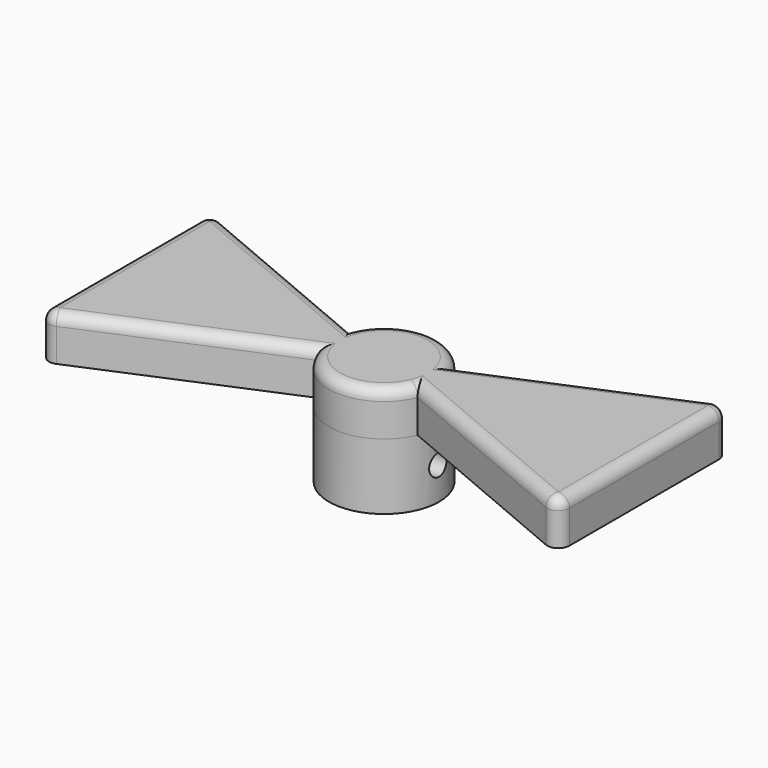
from build123d import *

# Parameters (mm, degrees)
F1_DEPTH      = 2
F2_R          = 2.5
F3_DEPTH      = 3
F4_R          = 0.5
F5_DEPTH      = 12.5
F6_T1_DEPTH   = 3.3861126193
F6_T3_DEPTH   = 8.4911099046
F6_T8_DEPTH   = 0.5
F6_T14_DEPTH  = 0.5
F6_T20_DEPTH  = 0.5
F6_T26_DEPTH  = 0.5
F6_T32_DEPTH  = 10.8279460436
F6_S33_R      = 2.5
F6_T34_DEPTH  = 7
F6_T36_ANGLE  = 134.1359227244
F6_T40_DEPTH  = 10.8279460436
F6_S41_R      = 2.5
F6_T42_DEPTH  = 7
F6_T46_DEPTH  = 10.8279460436
F6_S47_R      = 2.5
F6_T48_DEPTH  = 7
F6_T50_ANGLE  = 134.1359227244
F6_T54_DEPTH  = 10.8279460436
F6_S55_R      = 2.5
F6_T56_DEPTH  = 7
F6_T61_DEPTH  = 10.8279460436
F6_S62_R      = 2.5
F6_T63_DEPTH  = 7
F6_T66_ANGLE  = 162.8093840648
F6_T73_ANGLE  = 162.8093840648
F6_T77_DEPTH  = 10.8279460436
F6_S78_R      = 2.5
F6_T79_DEPTH  = 7
F6_T85_DEPTH  = 10.8279460436
F6_S86_R      = 2.5
F6_T87_DEPTH  = 7
F6_T90_ANGLE  = 162.8093840648
F6_T97_DEPTH  = 10.8279460436
F6_S98_R      = 2.5
F6_T99_DEPTH  = 7
F6_T102_ANGLE = 162.8093840648


# Not quite as in the source:
# - a fillet or chamfer that OpenCascade refuses, or shapes differently, is made with other operations: its cross-section is extruded or revolved along the edge and cut away or added


with BuildPart() as f1:
    # F0 (on Top) → F1 (new body)
    with BuildSketch(Plane.XY):
        with BuildLine():
            ThreePointArc((2.3024191783, -0.9740974937), (2.4501069309, -0.4969668269), (2.5, 0))
            ThreePointArc((2.5, 0), (2.4501069309, 0.4969668269), (2.3024191783, 0.9740974937))
            Line((2.3024191783, 0.9740974937), (0, 0))
            Line((0, 0), (2.3024191783, -0.9740974937))
        make_face()
        with BuildLine():
            ThreePointArc((2.3024191783, 0.9740974937), (2.4501069309, 0.4969668269), (2.5, 0))
            ThreePointArc((2.5, 0), (2.4501069309, -0.4969668269), (2.3024191783, -0.9740974937))
            Line((2.3024191783, -0.9740974937), (11.8182173411, -5))
            Line((11.8182173411, -5), (11.8182173411, 5))
            Line((11.8182173411, 5), (2.3024191783, 0.9740974937))
        make_face()
        with BuildLine():
            Line((0, 0), (2.3024191783, 0.9740974937))
            ThreePointArc((2.3024191783, 0.9740974937), (0, 2.5), (-2.3024191783, 0.9740974937))
            Line((-2.3024191783, 0.9740974937), (0, 0))
        make_face()
        with BuildLine():
            ThreePointArc((-2.3024191783, -0.9740974937), (0, -2.5), (2.3024191783, -0.9740974937))
            Line((2.3024191783, -0.9740974937), (0, 0))
            Line((0, 0), (-2.3024191783, -0.9740974937))
        make_face()
        with BuildLine():
            Line((0, 0), (-2.3024191783, 0.9740974937))
            ThreePointArc((-2.3024191783, 0.9740974937), (-2.5, 0), (-2.3024191783, -0.9740974937))
            Line((-2.3024191783, -0.9740974937), (0, 0))
        make_face()
        with BuildLine():
            ThreePointArc((-2.3024191783, -0.9740974937), (-2.5, 0), (-2.3024191783, 0.9740974937))
            Line((-2.3024191783, 0.9740974937), (-11.8182173411, 5))
            Line((-11.8182173411, 5), (-11.8182173411, -5))
            Line((-11.8182173411, -5), (-2.3024191783, -0.9740974937))
        make_face()
    extrude(amount=F1_DEPTH)

    # F2 (on face) → F3 (join)
    with BuildSketch(Plane(origin=(0, 0, 0), x_dir=(1, 0, 0), z_dir=(0, 0, -1))):
        Circle(F2_R)
    extrude(amount=F3_DEPTH)

    # F4 (on Right) → F5 (cut, symmetric)
    with BuildSketch(Plane.YZ):
        with Locations((0, -1.5)):
            Circle(F4_R)
    extrude(amount=F5_DEPTH, both=True, mode=Mode.SUBTRACT)

    # F6: fillet of radius 0.5 on 12 edges, made by hand

    # F6_s2 → F6_t1 (cut)
    with BuildSketch(Plane.XY.offset(-1.8861126193)):
        with BuildLine():
            ThreePointArc((-11.8182173411, -4.2455549523), (-11.5944330635, -4.6623341201), (-11.1233978424, -4.706038788))
            Line((-11.1233978424, -4.706038788), (-11.8182173411, -5))
            Line((-11.8182173411, -5), (-11.8182173411, -4.2455549523))
        make_face()
        with BuildLine():
            ThreePointArc((11.8182173411, 4.2455549523), (11.5944330635, 4.6623341201), (11.1233978424, 4.706038788))
            Line((11.1233978424, 4.706038788), (11.8182173411, 5))
            Line((11.8182173411, 5), (11.8182173411, 4.2455549523))
        make_face()
        with BuildLine():
            ThreePointArc((11.8182173411, -4.2455549523), (11.5944330635, -4.6623341201), (11.1233978424, -4.706038788))
            Line((11.1233978424, -4.706038788), (11.8182173411, -5))
            Line((11.8182173411, -5), (11.8182173411, -4.2455549523))
        make_face()
        with BuildLine():
            ThreePointArc((-11.1233978424, 4.706038788), (-11.5944330635, 4.6623341201), (-11.8182173411, 4.2455549523))
            Line((-11.8182173411, 4.2455549523), (-11.8182173411, 5))
            Line((-11.8182173411, 5), (-11.1233978424, 4.706038788))
        make_face()
    extrude(amount=F6_T1_DEPTH, mode=Mode.SUBTRACT)

    # F6_s4 → F6_t3 (cut)
    with BuildSketch(Plane.XZ.offset(-4.2455549523)):
        with BuildLine():
            ThreePointArc((11.8182173411, 1.5), (11.6717707317, 1.8535533906), (11.3182173411, 2))
            Line((11.3182173411, 2), (11.8182173411, 2))
            Line((11.8182173411, 2), (11.8182173411, 1.5))
        make_face()
        with BuildLine():
            ThreePointArc((-11.3182173411, 2), (-11.6717707317, 1.8535533906), (-11.8182173411, 1.5))
            Line((-11.8182173411, 1.5), (-11.8182173411, 2))
            Line((-11.8182173411, 2), (-11.3182173411, 2))
        make_face()
    extrude(amount=F6_T3_DEPTH, mode=Mode.SUBTRACT)


with BuildPart() as f6_tool6:
    # F6_s7 → F6_t8 (new body)
    with BuildSketch(Plane.XY.offset(1.5)):
        Polygon((-11.3182173411, -4.2455549523), (-11.8182173411, -4.2455549523), (-11.8182173411, -5), (-11.1233978424, -4.706038788), align=None)
    extrude(amount=F6_T8_DEPTH)

    # F6_s9 → F6_t10 (revolve, cut)
    with BuildSketch(Plane(origin=(-11.3182173411, -4.2455549523, 1.5), x_dir=(0.5524314449, 0.8335583355, 0), z_dir=(0.8335583355, -0.5524314449, 0))):
        with BuildLine():
            ThreePointArc((0, -0.5), (0.5, 0), (0, 0.5))
            Line((0, 0.5), (0, -0.5))
        make_face()
    revolve(axis=Axis((-11.3182173411, -4.2455549523, 1.5), (0, 0, 1)), mode=Mode.SUBTRACT)


with BuildPart() as f1_1:
    add(f1.part)

    # F6_t5: cut F6_tool6
    add(f6_tool6.part, mode=Mode.SUBTRACT)


with BuildPart() as f6_tool12:
    # F6_s13 → F6_t14 (new body)
    with BuildSketch(Plane.XY.offset(1.5)):
        Polygon((11.3182173411, 4.2455549523), (11.8182173411, 4.2455549523), (11.8182173411, 5), (11.1233978424, 4.706038788), align=None)
    extrude(amount=F6_T14_DEPTH)

    # F6_s15 → F6_t16 (revolve, cut)
    with BuildSketch(Plane(origin=(11.3182173411, 4.2455549523, 1.5), x_dir=(-0.5524314449, -0.8335583355, 0), z_dir=(-0.8335583355, 0.5524314449, 0))):
        with BuildLine():
            ThreePointArc((0, -0.5), (0.5, 0), (0, 0.5))
            Line((0, 0.5), (0, -0.5))
        make_face()
    revolve(axis=Axis((11.3182173411, 4.2455549523, 1.5), (0, 0, 1)), mode=Mode.SUBTRACT)


with BuildPart() as f1_2:
    add(f1_1.part)

    # F6_t11: cut F6_tool12
    add(f6_tool12.part, mode=Mode.SUBTRACT)


with BuildPart() as f6_tool18:
    # F6_s19 → F6_t20 (new body)
    with BuildSketch(Plane.XY.offset(1.5)):
        Polygon((11.3182173411, -4.2455549523), (11.8182173411, -4.2455549523), (11.8182173411, -5), (11.1233978424, -4.706038788), align=None)
    extrude(amount=F6_T20_DEPTH)

    # F6_s21 → F6_t22 (revolve, cut)
    with BuildSketch(Plane(origin=(11.3182173411, -4.2455549523, 1.5), x_dir=(-0.5524314449, 0.8335583355, 0), z_dir=(0.8335583355, 0.5524314449, 0))):
        with BuildLine():
            ThreePointArc((0, -0.5), (0.5, 0), (0, 0.5))
            Line((0, 0.5), (0, -0.5))
        make_face()
    revolve(axis=Axis((11.3182173411, -4.2455549523, 1.5), (0, 0, 1)), mode=Mode.SUBTRACT)


with BuildPart() as f1_3:
    add(f1_2.part)

    # F6_t17: cut F6_tool18
    add(f6_tool18.part, mode=Mode.SUBTRACT)


with BuildPart() as f6_tool24:
    # F6_s25 → F6_t26 (new body)
    with BuildSketch(Plane.XY.offset(1.5)):
        Polygon((-11.3182173411, 4.2455549523), (-11.1233978424, 4.706038788), (-11.8182173411, 5), (-11.8182173411, 4.2455549523), align=None)
    extrude(amount=F6_T26_DEPTH)

    # F6_s27 → F6_t28 (revolve, cut)
    with BuildSketch(Plane(origin=(-11.3182173411, 4.2455549523, 1.5), x_dir=(0.5524314449, -0.8335583355, 0), z_dir=(-0.8335583355, -0.5524314449, 0))):
        with BuildLine():
            ThreePointArc((0, -0.5), (0.5, 0), (0, 0.5))
            Line((0, 0.5), (0, -0.5))
        make_face()
    revolve(axis=Axis((-11.3182173411, 4.2455549523, 1.5), (0, 0, 1)), mode=Mode.SUBTRACT)


with BuildPart() as f1_4:
    add(f1_3.part)

    # F6_t23: cut F6_tool24
    add(f6_tool24.part, mode=Mode.SUBTRACT)


with BuildPart() as f6_tool30:
    # F6_s31 → F6_t32 (new body)
    with BuildSketch(Plane(origin=(11.1233978424, 4.706038788, 0), x_dir=(0, 0, 1), z_dir=(-0.9209676713, -0.3896389975, 0))):
        with BuildLine():
            ThreePointArc((1.5, 0), (1.8535533906, -0.1464466094), (2, -0.5))
            Line((2, -0.5), (2, 0))
            Line((2, 0), (1.5, 0))
        make_face()
    extrude(amount=F6_T32_DEPTH)

    # F6_s33 → F6_t34 (cut, symmetric)
    with BuildSketch(Plane.XY.offset(1.8)):
        Circle(F6_S33_R)
    extrude(amount=F6_T34_DEPTH, both=True, mode=Mode.SUBTRACT)


with BuildPart() as f1_5:
    add(f1_4.part)

    # F6_t29: cut F6_tool30
    add(f6_tool30.part, mode=Mode.SUBTRACT)

    # F6_s35 → F6_t36 (revolve, cut)
    with BuildSketch(Plane(origin=(0, 0, 0), x_dir=(0, 0, 1), z_dir=(0.3896389975, -0.9209676713, 0))):
        with BuildLine():
            ThreePointArc((2, -2), (1.8535533906, -2.3535533906), (1.5, -2.5))
            Line((1.5, -2.5), (2, -2.5))
            Line((2, -2.5), (2, -2))
        make_face()
    revolve(axis=Axis((0, 0, 2), (0, 0, 1)), revolution_arc=F6_T36_ANGLE, mode=Mode.SUBTRACT)


with BuildPart() as f6_tool38:
    # F6_s39 → F6_t40 (new body)
    with BuildSketch(Plane(origin=(-1.1512095892, 0.4870487468, 0), x_dir=(0, 0, 1), z_dir=(-0.9209676713, 0.3896389975, 0))):
        with BuildLine():
            ThreePointArc((2, -0.5), (1.8535533906, -0.1464466094), (1.5, 0))
            Line((1.5, 0), (2, 0))
            Line((2, 0), (2, -0.5))
        make_face()
    extrude(amount=F6_T40_DEPTH)

    # F6_s41 → F6_t42 (cut, symmetric)
    with BuildSketch(Plane.XY.offset(1.8)):
        Circle(F6_S41_R)
    extrude(amount=F6_T42_DEPTH, both=True, mode=Mode.SUBTRACT)


with BuildPart() as f1_6:
    add(f1_5.part)

    # F6_t37: cut F6_tool38
    add(f6_tool38.part, mode=Mode.SUBTRACT)


with BuildPart() as f6_tool44:
    # F6_s45 → F6_t46 (new body)
    with BuildSketch(Plane(origin=(-11.1233978424, -4.706038788, 0), x_dir=(0, 0, 1), z_dir=(0.9209676713, 0.3896389975, 0))):
        with BuildLine():
            ThreePointArc((2, -0.5), (1.8535533906, -0.1464466094), (1.5, 0))
            Line((1.5, 0), (2, 0))
            Line((2, 0), (2, -0.5))
        make_face()
    extrude(amount=F6_T46_DEPTH)

    # F6_s47 → F6_t48 (cut, symmetric)
    with BuildSketch(Plane.XY.offset(1.7)):
        Circle(F6_S47_R)
    extrude(amount=F6_T48_DEPTH, both=True, mode=Mode.SUBTRACT)


with BuildPart() as f1_7:
    add(f1_6.part)

    # F6_t43: cut F6_tool44
    add(f6_tool44.part, mode=Mode.SUBTRACT)

    # F6_s49 → F6_t50 (revolve, cut)
    with BuildSketch(Plane(origin=(0, 0, 0), x_dir=(0, 0, 1), z_dir=(-0.3896389975, 0.9209676713, 0))):
        with BuildLine():
            ThreePointArc((2, -2), (1.8535533906, -2.3535533906), (1.5, -2.5))
            Line((1.5, -2.5), (2, -2.5))
            Line((2, -2.5), (2, -2))
        make_face()
    revolve(axis=Axis((0, 0, 2), (0, 0, 1)), revolution_arc=F6_T50_ANGLE, mode=Mode.SUBTRACT)


with BuildPart() as f6_tool52:
    # F6_s53 → F6_t54 (new body)
    with BuildSketch(Plane(origin=(1.1512095892, -0.4870487468, 0), x_dir=(0, 0, 1), z_dir=(0.9209676713, -0.3896389975, 0))):
        with BuildLine():
            ThreePointArc((1.5, 0), (1.8535533906, -0.1464466094), (2, -0.5))
            Line((2, -0.5), (2, 0))
            Line((2, 0), (1.5, 0))
        make_face()
    extrude(amount=F6_T54_DEPTH)

    # F6_s55 → F6_t56 (cut, symmetric)
    with BuildSketch(Plane.XY.offset(1.8)):
        Circle(F6_S55_R)
    extrude(amount=F6_T56_DEPTH, both=True, mode=Mode.SUBTRACT)


with BuildPart() as f1_8:
    add(f1_7.part)

    # F6_t51: cut F6_tool52
    add(f6_tool52.part, mode=Mode.SUBTRACT)


with BuildPart() as f6_tool59:
    # F6_s60 → F6_t61 (new body)
    with BuildSketch(Plane(origin=(11.1233978424, 4.706038788, 0), x_dir=(0, 0, 1), z_dir=(-0.9209676713, -0.3896389975, 0))):
        with BuildLine():
            ThreePointArc((1.5, 0), (1.8535533906, -0.1464466094), (2, -0.5))
            Line((2, -0.5), (2, 0))
            Line((2, 0), (1.5, 0))
        make_face()
    extrude(amount=F6_T61_DEPTH)

    # F6_s62 → F6_t63 (intersect, symmetric)
    with BuildSketch(Plane.XY.offset(1.8)):
        Circle(F6_S62_R)
    extrude(amount=F6_T63_DEPTH, both=True, mode=Mode.INTERSECT)


with BuildPart() as f6_tool64:
    # F6_s65 → F6_t66 (revolve)
    with BuildSketch(Plane(origin=(0, 0, 0), x_dir=(0, 0, 1), z_dir=(-0.1000391116, -0.9949835055, 0))):
        with BuildLine():
            ThreePointArc((2, -2), (1.8535533906, -2.3535533906), (1.5, -2.5))
            Line((1.5, -2.5), (2, -2.5))
            Line((2, -2.5), (2, -2))
        make_face()
    revolve(axis=Axis((0, 0, 2), (0, 0, 1)), revolution_arc=F6_T66_ANGLE)

    split(bisect_by=Plane(origin=(0, 0, 0), x_dir=(0, 0, 1), z_dir=(0.3896389975, -0.9209676713, 0)), keep=Keep.TOP)


with BuildPart() as f6_tool59_1:
    add(f6_tool59.part)

    # F6_t68: intersect F6_tool64
    add(f6_tool64.part, mode=Mode.INTERSECT)


with BuildPart() as f1_9:
    add(f1_8.part)

    # F6_t57: cut F6_tool59
    add(f6_tool59_1.part, mode=Mode.SUBTRACT)


with BuildPart() as f6_tool71:
    # F6_s72 → F6_t73 (revolve)
    with BuildSketch(Plane(origin=(0, 0, 0), x_dir=(0, 0, 1), z_dir=(0.3896389975, -0.9209676713, 0))):
        with BuildLine():
            ThreePointArc((2, -2), (1.8535533906, -2.3535533906), (1.5, -2.5))
            Line((1.5, -2.5), (2, -2.5))
            Line((2, -2.5), (2, -2))
        make_face()
    revolve(axis=Axis((0, 0, 2), (0, 0, 1)), revolution_arc=F6_T73_ANGLE)

    split(bisect_by=Plane(origin=(0, 0, 0), x_dir=(0, 0, 1), z_dir=(-0.3896389975, -0.9209676713, 0)), keep=Keep.TOP)


with BuildPart() as f6_tool75:
    # F6_s76 → F6_t77 (new body)
    with BuildSketch(Plane(origin=(-1.1512095892, 0.4870487468, 0), x_dir=(0, 0, 1), z_dir=(-0.9209676713, 0.3896389975, 0))):
        with BuildLine():
            ThreePointArc((2, -0.5), (1.8535533906, -0.1464466094), (1.5, 0))
            Line((1.5, 0), (2, 0))
            Line((2, 0), (2, -0.5))
        make_face()
    extrude(amount=F6_T77_DEPTH)

    # F6_s78 → F6_t79 (intersect, symmetric)
    with BuildSketch(Plane.XY.offset(1.8)):
        Circle(F6_S78_R)
    extrude(amount=F6_T79_DEPTH, both=True, mode=Mode.INTERSECT)


with BuildPart() as f6_tool71_1:
    add(f6_tool71.part)

    # F6_t80: intersect F6_tool75
    add(f6_tool75.part, mode=Mode.INTERSECT)


with BuildPart() as f1_10:
    add(f1_9.part)

    # F6_t69: cut F6_tool71
    add(f6_tool71_1.part, mode=Mode.SUBTRACT)


with BuildPart() as f6_tool83:
    # F6_s84 → F6_t85 (new body)
    with BuildSketch(Plane(origin=(-11.1233978424, -4.706038788, 0), x_dir=(0, 0, 1), z_dir=(0.9209676713, 0.3896389975, 0))):
        with BuildLine():
            ThreePointArc((2, -0.5), (1.8535533906, -0.1464466094), (1.5, 0))
            Line((1.5, 0), (2, 0))
            Line((2, 0), (2, -0.5))
        make_face()
    extrude(amount=F6_T85_DEPTH)

    # F6_s86 → F6_t87 (intersect, symmetric)
    with BuildSketch(Plane.XY.offset(1.7)):
        Circle(F6_S86_R)
    extrude(amount=F6_T87_DEPTH, both=True, mode=Mode.INTERSECT)


with BuildPart() as f6_tool88:
    # F6_s89 → F6_t90 (revolve)
    with BuildSketch(Plane(origin=(0, 0, 0), x_dir=(0, 0, 1), z_dir=(0.1000391116, 0.9949835055, 0))):
        with BuildLine():
            ThreePointArc((2, -2), (1.8535533906, -2.3535533906), (1.5, -2.5))
            Line((1.5, -2.5), (2, -2.5))
            Line((2, -2.5), (2, -2))
        make_face()
    revolve(axis=Axis((0, 0, 2), (0, 0, 1)), revolution_arc=F6_T90_ANGLE)

    split(bisect_by=Plane(origin=(0, 0, 0), x_dir=(0, 0, 1), z_dir=(-0.3896389975, 0.9209676713, 0)), keep=Keep.TOP)


with BuildPart() as f6_tool83_1:
    add(f6_tool83.part)

    # F6_t92: intersect F6_tool88
    add(f6_tool88.part, mode=Mode.INTERSECT)


with BuildPart() as f1_11:
    add(f1_10.part)

    # F6_t81: cut F6_tool83
    add(f6_tool83_1.part, mode=Mode.SUBTRACT)


with BuildPart() as f6_tool95:
    # F6_s96 → F6_t97 (new body)
    with BuildSketch(Plane(origin=(1.1512095892, -0.4870487468, 0), x_dir=(0, 0, 1), z_dir=(0.9209676713, -0.3896389975, 0))):
        with BuildLine():
            ThreePointArc((1.5, 0), (1.8535533906, -0.1464466094), (2, -0.5))
            Line((2, -0.5), (2, 0))
            Line((2, 0), (1.5, 0))
        make_face()
    extrude(amount=F6_T97_DEPTH)

    # F6_s98 → F6_t99 (intersect, symmetric)
    with BuildSketch(Plane.XY.offset(1.8)):
        Circle(F6_S98_R)
    extrude(amount=F6_T99_DEPTH, both=True, mode=Mode.INTERSECT)


with BuildPart() as f6_tool100:
    # F6_s101 → F6_t102 (revolve)
    with BuildSketch(Plane(origin=(0, 0, 0), x_dir=(0, 0, 1), z_dir=(-0.3896389975, 0.9209676713, 0))):
        with BuildLine():
            ThreePointArc((2, -2), (1.8535533906, -2.3535533906), (1.5, -2.5))
            Line((1.5, -2.5), (2, -2.5))
            Line((2, -2.5), (2, -2))
        make_face()
    revolve(axis=Axis((0, 0, 2), (0, 0, 1)), revolution_arc=F6_T102_ANGLE)

    split(bisect_by=Plane(origin=(0, 0, 0), x_dir=(0, 0, 1), z_dir=(0.3896389975, 0.9209676713, 0)), keep=Keep.TOP)


with BuildPart() as f6_tool95_1:
    add(f6_tool95.part)

    # F6_t104: intersect F6_tool100
    add(f6_tool100.part, mode=Mode.INTERSECT)


with BuildPart() as f1_12:
    add(f1_11.part)

    # F6_t93: cut F6_tool95
    add(f6_tool95_1.part, mode=Mode.SUBTRACT)


solid = f1_12.part
